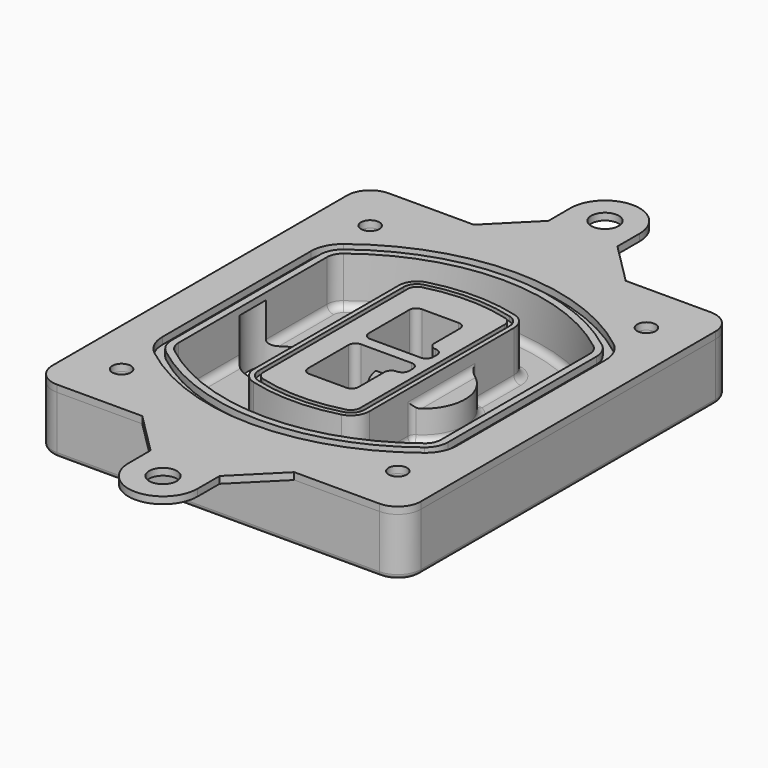
from build123d import *

# Parameters (mm, degrees)
F0_R      = 4
F1_DEPTH  = 25
F2_DEPTH  = 3
F3_DEPTH  = 18
F5_DEPTH  = 21
F6_DEPTH  = 2
F8_DEPTH  = 20
F9_DEPTH  = 16
F10_DEPTH = 25
F7_R      = 6
F7_R_2    = 4
F11_DEPTH = 6
F13_DEPTH = 9
F14_R     = 3
F15_R     = 2
F16_R     = 6
F16_R_2   = 4
F17_DEPTH = 3


with BuildPart() as f1:
    # F0 (on Top) → F1 (new body)
    with BuildSketch(Plane.XY):
        with BuildLine():
            ThreePointArc((-80, -80), (-77.0710678119, -87.0710678119), (-70, -90))
            Line((-70, -90), (70, -90))
            ThreePointArc((70, -90), (77.0710678119, -87.0710678119), (80, -80))
            Line((80, -80), (80, 80))
            ThreePointArc((80, 80), (77.0710678119, 87.0710678119), (70, 90))
            Line((70, 90), (-70, 90))
            ThreePointArc((-70, 90), (-77.0710678119, 87.0710678119), (-80, 80))
            Line((-80, 80), (-80, -80))
        make_face()
        with Locations((-60, -67.5)):
            Circle(F0_R, mode=Mode.SUBTRACT)
        with Locations((60, -67.5)):
            Circle(F0_R, mode=Mode.SUBTRACT)
        with Locations((-60, 67.5)):
            Circle(F0_R, mode=Mode.SUBTRACT)
        with BuildLine():
            ThreePointArc((-64, 40.2934422872), (-62.5820384798, 46.4328484224), (-58.6153846154, 51.3286200352))
            ThreePointArc((-58.6153846154, 51.3286200352), (0, 71.5), (58.6153846154, 51.3286200352))
            ThreePointArc((58.6153846154, 51.3286200352), (62.5820384798, 46.4328484224), (64, 40.2934422872))
            Line((64, 40.2934422872), (64, -40.2934422872))
            ThreePointArc((64, -40.2934422872), (62.5820384798, -46.4328484224), (58.6153846154, -51.3286200352))
            ThreePointArc((58.6153846154, -51.3286200352), (0, -71.5), (-58.6153846154, -51.3286200352))
            ThreePointArc((-58.6153846154, -51.3286200352), (-62.5820384798, -46.4328484224), (-64, -40.2934422872))
            Line((-64, -40.2934422872), (-64, 40.2934422872))
        make_face(mode=Mode.SUBTRACT)
        with Locations((60, 67.5)):
            Circle(F0_R, mode=Mode.SUBTRACT)
        with BuildLine():
            ThreePointArc((58.6153846154, 51.3286200352), (0, 71.5), (-58.6153846154, 51.3286200352))
            ThreePointArc((-58.6153846154, 51.3286200352), (-62.5820384798, 46.4328484224), (-64, 40.2934422872))
            Line((-64, 40.2934422872), (-64, -40.2934422872))
            ThreePointArc((-64, -40.2934422872), (-62.5820384798, -46.4328484224), (-58.6153846154, -51.3286200352))
            ThreePointArc((-58.6153846154, -51.3286200352), (0, -71.5), (58.6153846154, -51.3286200352))
            ThreePointArc((58.6153846154, -51.3286200352), (62.5820384798, -46.4328484224), (64, -40.2934422872))
            Line((64, -40.2934422872), (64, 40.2934422872))
            ThreePointArc((64, 40.2934422872), (62.5820384798, 46.4328484224), (58.6153846154, 51.3286200352))
        make_face()
        with BuildLine():
            Line((-60, -40.2934422872), (-60, 40.2934422872))
            ThreePointArc((-60, 40.2934422872), (-58.9871703427, 44.6787323838), (-56.1538461538, 48.1757121072))
            ThreePointArc((-56.1538461538, 48.1757121072), (0, 67.5), (56.1538461538, 48.1757121072))
            ThreePointArc((56.1538461538, 48.1757121072), (58.9871703427, 44.6787323838), (60, 40.2934422872))
            Line((60, 40.2934422872), (60, -40.2934422872))
            ThreePointArc((60, -40.2934422872), (58.9871703427, -44.6787323838), (56.1538461538, -48.1757121072))
            ThreePointArc((56.1538461538, -48.1757121072), (0, -67.5), (-56.1538461538, -48.1757121072))
            ThreePointArc((-56.1538461538, -48.1757121072), (-58.9871703427, -44.6787323838), (-60, -40.2934422872))
        make_face(mode=Mode.SUBTRACT)
        with BuildLine():
            ThreePointArc((-56.1538461538, 48.1757121072), (-58.9871703427, 44.6787323838), (-60, 40.2934422872))
            Line((-60, 40.2934422872), (-60, -40.2934422872))
            ThreePointArc((-60, -40.2934422872), (-58.9871703427, -44.6787323838), (-56.1538461538, -48.1757121072))
            ThreePointArc((-56.1538461538, -48.1757121072), (0, -67.5), (56.1538461538, -48.1757121072))
            ThreePointArc((56.1538461538, -48.1757121072), (58.9871703427, -44.6787323838), (60, -40.2934422872))
            Line((60, -40.2934422872), (60, 40.2934422872))
            ThreePointArc((60, 40.2934422872), (58.9871703427, 44.6787323838), (56.1538461538, 48.1757121072))
            ThreePointArc((56.1538461538, 48.1757121072), (0, 67.5), (-56.1538461538, 48.1757121072))
        make_face()
        with BuildLine():
            ThreePointArc((54.3076923077, 45.8110311612), (56.2910192399, 43.3631453548), (57, 40.2934422872))
            Line((57, 40.2934422872), (57, -40.2934422872))
            ThreePointArc((57, -40.2934422872), (56.2910192399, -43.3631453548), (54.3076923077, -45.8110311612))
            ThreePointArc((54.3076923077, -45.8110311612), (0, -64.5), (-54.3076923077, -45.8110311612))
            ThreePointArc((-54.3076923077, -45.8110311612), (-56.2910192399, -43.3631453548), (-57, -40.2934422872))
            Line((-57, -40.2934422872), (-57, 40.2934422872))
            ThreePointArc((-57, 40.2934422872), (-56.2910192399, 43.3631453548), (-54.3076923077, 45.8110311612))
            ThreePointArc((-54.3076923077, 45.8110311612), (0, 64.5), (54.3076923077, 45.8110311612))
        make_face(mode=Mode.SUBTRACT)
        with BuildLine():
            Line((57, -40.2934422872), (57, 40.2934422872))
            ThreePointArc((57, 40.2934422872), (56.2910192399, 43.3631453548), (54.3076923077, 45.8110311612))
            ThreePointArc((54.3076923077, 45.8110311612), (0, 64.5), (-54.3076923077, 45.8110311612))
            ThreePointArc((-54.3076923077, 45.8110311612), (-56.2910192399, 43.3631453548), (-57, 40.2934422872))
            Line((-57, 40.2934422872), (-57, -40.2934422872))
            ThreePointArc((-57, -40.2934422872), (-56.2910192399, -43.3631453548), (-54.3076923077, -45.8110311612))
            ThreePointArc((-54.3076923077, -45.8110311612), (0, -64.5), (54.3076923077, -45.8110311612))
            ThreePointArc((54.3076923077, -45.8110311612), (56.2910192399, -43.3631453548), (57, -40.2934422872))
        make_face()
    extrude(amount=-F1_DEPTH)

    # F0 (on Top) → F2 (join)
    with BuildSketch(Plane.XY):
        with BuildLine():
            ThreePointArc((-56.1538461538, 48.1757121072), (-58.9871703427, 44.6787323838), (-60, 40.2934422872))
            Line((-60, 40.2934422872), (-60, -40.2934422872))
            ThreePointArc((-60, -40.2934422872), (-58.9871703427, -44.6787323838), (-56.1538461538, -48.1757121072))
            ThreePointArc((-56.1538461538, -48.1757121072), (0, -67.5), (56.1538461538, -48.1757121072))
            ThreePointArc((56.1538461538, -48.1757121072), (58.9871703427, -44.6787323838), (60, -40.2934422872))
            Line((60, -40.2934422872), (60, 40.2934422872))
            ThreePointArc((60, 40.2934422872), (58.9871703427, 44.6787323838), (56.1538461538, 48.1757121072))
            ThreePointArc((56.1538461538, 48.1757121072), (0, 67.5), (-56.1538461538, 48.1757121072))
        make_face()
        with BuildLine():
            ThreePointArc((54.3076923077, 45.8110311612), (56.2910192399, 43.3631453548), (57, 40.2934422872))
            Line((57, 40.2934422872), (57, -40.2934422872))
            ThreePointArc((57, -40.2934422872), (56.2910192399, -43.3631453548), (54.3076923077, -45.8110311612))
            ThreePointArc((54.3076923077, -45.8110311612), (0, -64.5), (-54.3076923077, -45.8110311612))
            ThreePointArc((-54.3076923077, -45.8110311612), (-56.2910192399, -43.3631453548), (-57, -40.2934422872))
            Line((-57, -40.2934422872), (-57, 40.2934422872))
            ThreePointArc((-57, 40.2934422872), (-56.2910192399, 43.3631453548), (-54.3076923077, 45.8110311612))
            ThreePointArc((-54.3076923077, 45.8110311612), (0, 64.5), (54.3076923077, 45.8110311612))
        make_face(mode=Mode.SUBTRACT)
    extrude(amount=F2_DEPTH)

    # F0 (on Top) → F3 (cut)
    with BuildSketch(Plane.XY):
        with BuildLine():
            Line((57, -40.2934422872), (57, 40.2934422872))
            ThreePointArc((57, 40.2934422872), (56.2910192399, 43.3631453548), (54.3076923077, 45.8110311612))
            ThreePointArc((54.3076923077, 45.8110311612), (0, 64.5), (-54.3076923077, 45.8110311612))
            ThreePointArc((-54.3076923077, 45.8110311612), (-56.2910192399, 43.3631453548), (-57, 40.2934422872))
            Line((-57, 40.2934422872), (-57, -40.2934422872))
            ThreePointArc((-57, -40.2934422872), (-56.2910192399, -43.3631453548), (-54.3076923077, -45.8110311612))
            ThreePointArc((-54.3076923077, -45.8110311612), (0, -64.5), (54.3076923077, -45.8110311612))
            ThreePointArc((54.3076923077, -45.8110311612), (56.2910192399, -43.3631453548), (57, -40.2934422872))
        make_face()
    extrude(amount=-F3_DEPTH, mode=Mode.SUBTRACT)

    # F4 (on face) → F5 (join, through all)
    with BuildSketch(Plane.XY.offset(3)):
        with BuildLine():
            ThreePointArc((-25, -39.2465276821), (-23.3511545998, -44.1109737193), (-19.0842911877, -46.9702398883))
            ThreePointArc((-19.0842911877, -46.9702398883), (0, -49.5), (19.0842911877, -46.9702398883))
            ThreePointArc((19.0842911877, -46.9702398883), (23.3511545998, -44.1109737193), (25, -39.2465276821))
            Line((25, -39.2465276821), (25, 39.2465276821))
            ThreePointArc((25, 39.2465276821), (23.3511545998, 44.1109737193), (19.0842911877, 46.9702398883))
            ThreePointArc((19.0842911877, 46.9702398883), (0, 49.5), (-19.0842911877, 46.9702398883))
            ThreePointArc((-19.0842911877, 46.9702398883), (-23.3511545998, 44.1109737193), (-25, 39.2465276821))
            Line((-25, 39.2465276821), (-25, -39.2465276821))
        make_face()
        with BuildLine():
            ThreePointArc((18.5632183908, 45.0393118368), (21.7633659499, 42.89486221), (23, 39.2465276821))
            Line((23, 39.2465276821), (23, -39.2465276821))
            ThreePointArc((23, -39.2465276821), (21.7633659499, -42.89486221), (18.5632183908, -45.0393118368))
            ThreePointArc((18.5632183908, -45.0393118368), (0, -47.5), (-18.5632183908, -45.0393118368))
            ThreePointArc((-18.5632183908, -45.0393118368), (-21.7633659499, -42.89486221), (-23, -39.2465276821))
            Line((-23, -39.2465276821), (-23, 39.2465276821))
            ThreePointArc((-23, 39.2465276821), (-21.7633659499, 42.89486221), (-18.5632183908, 45.0393118368))
            ThreePointArc((-18.5632183908, 45.0393118368), (0, 47.5), (18.5632183908, 45.0393118368))
        make_face(mode=Mode.SUBTRACT)
        with BuildLine():
            Line((23, -39.2465276821), (23, 39.2465276821))
            ThreePointArc((23, 39.2465276821), (21.7633659499, 42.89486221), (18.5632183908, 45.0393118368))
            ThreePointArc((18.5632183908, 45.0393118368), (0, 47.5), (-18.5632183908, 45.0393118368))
            ThreePointArc((-18.5632183908, 45.0393118368), (-21.7633659499, 42.89486221), (-23, 39.2465276821))
            Line((-23, 39.2465276821), (-23, -39.2465276821))
            ThreePointArc((-23, -39.2465276821), (-21.7633659499, -42.89486221), (-18.5632183908, -45.0393118368))
            ThreePointArc((-18.5632183908, -45.0393118368), (0, -47.5), (18.5632183908, -45.0393118368))
            ThreePointArc((18.5632183908, -45.0393118368), (21.7633659499, -42.89486221), (23, -39.2465276821))
        make_face()
        with BuildLine():
            ThreePointArc((18.0421455939, 43.1083837852), (20.1755772999, 41.6787507007), (21, 39.2465276821))
            Line((21, 39.2465276821), (21, -39.2465276821))
            ThreePointArc((21, -39.2465276821), (20.1755772999, -41.6787507007), (18.0421455939, -43.1083837852))
            ThreePointArc((18.0421455939, -43.1083837852), (0, -45.5), (-18.0421455939, -43.1083837852))
            ThreePointArc((-18.0421455939, -43.1083837852), (-20.1755772999, -41.6787507007), (-21, -39.2465276821))
            Line((-21, -39.2465276821), (-21, 39.2465276821))
            ThreePointArc((-21, 39.2465276821), (-20.1755772999, 41.6787507007), (-18.0421455939, 43.1083837852))
            ThreePointArc((-18.0421455939, 43.1083837852), (0, 45.5), (18.0421455939, 43.1083837852))
        make_face(mode=Mode.SUBTRACT)
        with BuildLine():
            Line((21, -39.2465276821), (21, 39.2465276821))
            ThreePointArc((21, 39.2465276821), (20.1755772999, 41.6787507007), (18.0421455939, 43.1083837852))
            ThreePointArc((18.0421455939, 43.1083837852), (0, 45.5), (-18.0421455939, 43.1083837852))
            ThreePointArc((-18.0421455939, 43.1083837852), (-20.1755772999, 41.6787507007), (-21, 39.2465276821))
            Line((-21, 39.2465276821), (-21, -39.2465276821))
            ThreePointArc((-21, -39.2465276821), (-20.1755772999, -41.6787507007), (-18.0421455939, -43.1083837852))
            ThreePointArc((-18.0421455939, -43.1083837852), (0, -45.5), (18.0421455939, -43.1083837852))
            ThreePointArc((18.0421455939, -43.1083837852), (20.1755772999, -41.6787507007), (21, -39.2465276821))
        make_face()
        with BuildLine():
            Line((-8, -2.5), (14, -2.5))
            ThreePointArc((14, -2.5), (16.1213203436, -3.3786796564), (17, -5.5))
            Line((17, -5.5), (17, -7.5))
            ThreePointArc((17, -7.5), (16.1213203436, -9.6213203436), (14, -10.5))
            ThreePointArc((14, -10.5), (11.8786796564, -11.3786796564), (11, -13.5))
            Line((11, -13.5), (11, -27.5))
            ThreePointArc((11, -27.5), (10.1213203436, -29.6213203436), (8, -30.5))
            Line((8, -30.5), (-8, -30.5))
            ThreePointArc((-8, -30.5), (-10.1213203436, -29.6213203436), (-11, -27.5))
            Line((-11, -27.5), (-11, -5.5))
            ThreePointArc((-11, -5.5), (-10.1213203436, -3.3786796564), (-8, -2.5))
        make_face(mode=Mode.SUBTRACT)
        with BuildLine():
            ThreePointArc((-8, 2.5), (-10.1213203436, 3.3786796564), (-11, 5.5))
            Line((-11, 5.5), (-11, 27.5))
            ThreePointArc((-11, 27.5), (-10.1213203436, 29.6213203436), (-8, 30.5))
            Line((-8, 30.5), (8, 30.5))
            ThreePointArc((8, 30.5), (10.1213203436, 29.6213203436), (11, 27.5))
            Line((11, 27.5), (11, 13.5))
            ThreePointArc((11, 13.5), (11.8786796564, 11.3786796564), (14, 10.5))
            ThreePointArc((14, 10.5), (16.1213203436, 9.6213203436), (17, 7.5))
            Line((17, 7.5), (17, 5.5))
            ThreePointArc((17, 5.5), (16.1213203436, 3.3786796564), (14, 2.5))
            Line((14, 2.5), (-8, 2.5))
        make_face(mode=Mode.SUBTRACT)
    extrude(amount=-F5_DEPTH)

    # F4 (on face) → F6 (cut)
    with BuildSketch(Plane.XY.offset(3)):
        with BuildLine():
            Line((23, -39.2465276821), (23, 39.2465276821))
            ThreePointArc((23, 39.2465276821), (21.7633659499, 42.89486221), (18.5632183908, 45.0393118368))
            ThreePointArc((18.5632183908, 45.0393118368), (0, 47.5), (-18.5632183908, 45.0393118368))
            ThreePointArc((-18.5632183908, 45.0393118368), (-21.7633659499, 42.89486221), (-23, 39.2465276821))
            Line((-23, 39.2465276821), (-23, -39.2465276821))
            ThreePointArc((-23, -39.2465276821), (-21.7633659499, -42.89486221), (-18.5632183908, -45.0393118368))
            ThreePointArc((-18.5632183908, -45.0393118368), (0, -47.5), (18.5632183908, -45.0393118368))
            ThreePointArc((18.5632183908, -45.0393118368), (21.7633659499, -42.89486221), (23, -39.2465276821))
        make_face()
        with BuildLine():
            ThreePointArc((18.0421455939, 43.1083837852), (20.1755772999, 41.6787507007), (21, 39.2465276821))
            Line((21, 39.2465276821), (21, -39.2465276821))
            ThreePointArc((21, -39.2465276821), (20.1755772999, -41.6787507007), (18.0421455939, -43.1083837852))
            ThreePointArc((18.0421455939, -43.1083837852), (0, -45.5), (-18.0421455939, -43.1083837852))
            ThreePointArc((-18.0421455939, -43.1083837852), (-20.1755772999, -41.6787507007), (-21, -39.2465276821))
            Line((-21, -39.2465276821), (-21, 39.2465276821))
            ThreePointArc((-21, 39.2465276821), (-20.1755772999, 41.6787507007), (-18.0421455939, 43.1083837852))
            ThreePointArc((-18.0421455939, 43.1083837852), (0, 45.5), (18.0421455939, 43.1083837852))
        make_face(mode=Mode.SUBTRACT)
    extrude(amount=-F6_DEPTH, mode=Mode.SUBTRACT)

    # F7 (on face) → F8 (join)
    with BuildSketch(Plane(origin=(0, 0, -25), x_dir=(1, 0, 0), z_dir=(0, 0, -1))):
        with BuildLine():
            ThreePointArc((3.28842436, 0), (16.7567035675, 13.4682792075), (30.224982775, 0))
            Line((30.224982775, 0), (35.224982775, 0))
            ThreePointArc((35.224982775, 0), (16.7567035675, 18.4682792075), (-1.71157564, 0))
            Line((-1.71157564, 0), (3.28842436, 0))
        make_face()
        with BuildLine():
            Line((3.28842436, 0), (30.224982775, 0))
            ThreePointArc((30.224982775, 0), (16.7567035675, 13.4682792075), (3.28842436, 0))
        make_face()
        with BuildLine():
            ThreePointArc((3.28842436, 0), (16.7567035675, -13.4682792075), (30.224982775, 0))
            Line((30.224982775, 0), (3.28842436, 0))
        make_face()
        with BuildLine():
            Line((35.224982775, 0), (30.224982775, 0))
            ThreePointArc((30.224982775, 0), (16.7567035675, -13.4682792075), (3.28842436, 0))
            Line((3.28842436, 0), (-1.71157564, 0))
            ThreePointArc((-1.71157564, 0), (16.7567035675, -18.4682792075), (35.224982775, 0))
        make_face()
    extrude(amount=-F8_DEPTH)

    # F7 (on face) → F9 (cut)
    with BuildSketch(Plane(origin=(0, 0, -25), x_dir=(1, 0, 0), z_dir=(0, 0, -1))):
        with BuildLine():
            Line((3.28842436, 0), (30.224982775, 0))
            ThreePointArc((30.224982775, 0), (16.7567035675, 13.4682792075), (3.28842436, 0))
        make_face()
        with BuildLine():
            ThreePointArc((3.28842436, 0), (16.7567035675, -13.4682792075), (30.224982775, 0))
            Line((30.224982775, 0), (3.28842436, 0))
        make_face()
    extrude(amount=-F9_DEPTH, mode=Mode.SUBTRACT)

    # F7 (on face) → F10 (cut)
    with BuildSketch(Plane(origin=(0, 0, -25), x_dir=(1, 0, 0), z_dir=(0, 0, -1))):
        with BuildLine():
            Line((-59.0318229325, 0), (-32.0952645175, 0))
            ThreePointArc((-32.0952645175, 0), (-45.563543725, 13.4682792075), (-59.0318229325, 0))
        make_face()
        with BuildLine():
            ThreePointArc((-59.0318229325, 0), (-45.563543725, -13.4682792075), (-32.0952645175, 0))
            Line((-32.0952645175, 0), (-59.0318229325, 0))
        make_face()
    extrude(amount=-F10_DEPTH, mode=Mode.SUBTRACT)

    # F7 (on face) → F11 (cut)
    with BuildSketch(Plane(origin=(0, 0, -25), x_dir=(1, 0, 0), z_dir=(0, 0, -1))):
        with Locations((60, -67.5)):
            Circle(F7_R)
        with Locations((60, -67.5)):
            Circle(F7_R_2, mode=Mode.SUBTRACT)
        with Locations((-60, -67.5)):
            Circle(F7_R)
        with Locations((-60, -67.5)):
            Circle(F7_R_2, mode=Mode.SUBTRACT)
        with Locations((-60, 67.5)):
            Circle(F7_R)
        with Locations((-60, 67.5)):
            Circle(F7_R_2, mode=Mode.SUBTRACT)
        with Locations((60, 67.5)):
            Circle(F7_R)
        with Locations((60, 67.5)):
            Circle(F7_R_2, mode=Mode.SUBTRACT)
    extrude(amount=-F11_DEPTH, mode=Mode.SUBTRACT)

    # F12 (on face) → F13 (cut, through all)
    with BuildSketch(Plane(origin=(0, 0, -9), x_dir=(1, 0, 0), z_dir=(0, 0, -1))):
        with BuildLine():
            Line((11, 13.5), (11, 17.5481537753))
            ThreePointArc((11, 17.5481537753), (2.5696536419, 11.8239143813), (-1.5415842455, 2.5))
            Line((-1.5415842455, 2.5), (3.5224848595, 2.5))
            ThreePointArc((3.5224848595, 2.5), (6.1857188154, 8.3455872281), (11.2536447004, 12.2927168648))
            ThreePointArc((11.2536447004, 12.2927168648), (11.0640958889, 12.8831798879), (11, 13.5))
        make_face()
        with BuildLine():
            ThreePointArc((11.2536447004, -12.2927168648), (6.1857188154, -8.3455872281), (3.5224848595, -2.5))
            Line((3.5224848595, -2.5), (-1.5415842455, -2.5))
            ThreePointArc((-1.5415842455, -2.5), (2.5696536419, -11.8239143813), (11, -17.5481537753))
            Line((11, -17.5481537753), (11, -13.5))
            ThreePointArc((11, -13.5), (11.0640958889, -12.8831798879), (11.2536447004, -12.2927168648))
        make_face()
        with BuildLine():
            ThreePointArc((11.2536447004, 12.2927168648), (6.1857188154, 8.3455872281), (3.5224848595, 2.5))
            Line((3.5224848595, 2.5), (14, 2.5))
            ThreePointArc((14, 2.5), (16.1213203436, 3.3786796564), (17, 5.5))
            Line((17, 5.5), (17, 7.5))
            ThreePointArc((17, 7.5), (16.1213203436, 9.6213203436), (14, 10.5))
            ThreePointArc((14, 10.5), (12.3601599782, 10.9878446101), (11.2536447004, 12.2927168648))
        make_face()
        with BuildLine():
            Line((14, -2.5), (3.5224848595, -2.5))
            ThreePointArc((3.5224848595, -2.5), (6.1857188154, -8.3455872281), (11.2536447004, -12.2927168648))
            ThreePointArc((11.2536447004, -12.2927168648), (12.3601599782, -10.9878446101), (14, -10.5))
            ThreePointArc((14, -10.5), (16.1213203436, -9.6213203436), (17, -7.5))
            Line((17, -7.5), (17, -5.5))
            ThreePointArc((17, -5.5), (16.1213203436, -3.3786796564), (14, -2.5))
        make_face()
    extrude(amount=F13_DEPTH, mode=Mode.SUBTRACT)

    # F14
    f14_edges = [f1.edges().sort_by_distance(p)[0] for p in [
        (-57, -23.703476, -18),
        (-57, 23.703476, -18),
        (25, 0, -5),
        (25, 16.526506, -11.5),
        (25, -16.526506, -11.5),
        (25, -27.886517, -18),
        (35.224983, 0, -18),
    ]]
    fillet(f14_edges, radius=F14_R)

    # F15
    f15_edges = [f1.edges().sort_by_distance(p)[0] for p in [
        (0, -90, -25),
    ]]
    fillet(f15_edges, radius=F15_R)


with BuildPart() as f17:
    # F16 (on face) → F17 (new body, through all)
    with BuildSketch(Plane.XY):
        with BuildLine():
            Line((33, -90), (-33, -90))
            Line((-33, -90), (-15, -108))
            Line((-15, -108), (-15, -120))
            ThreePointArc((-15, -120), (0, -135), (15, -120))
            Line((15, -120), (15, -108))
            Line((15, -108), (33, -90))
        make_face()
        with Locations((0, -120)):
            Circle(F16_R, mode=Mode.SUBTRACT)
        with BuildLine():
            Line((33, 90), (-33, 90))
            Line((-33, 90), (-70, 90))
            ThreePointArc((-70, 90), (-77.0710678119, 87.0710678119), (-80, 80))
            Line((-80, 80), (-80, -80))
            ThreePointArc((-80, -80), (-77.0710678119, -87.0710678119), (-70, -90))
            Line((-70, -90), (-33, -90))
            Line((-33, -90), (33, -90))
            Line((33, -90), (70, -90))
            ThreePointArc((70, -90), (77.0710678119, -87.0710678119), (80, -80))
            Line((80, -80), (80, 80))
            ThreePointArc((80, 80), (77.0710678119, 87.0710678119), (70, 90))
            Line((70, 90), (33, 90))
        make_face()
        with Locations((-60, -67.5)):
            Circle(F16_R_2, mode=Mode.SUBTRACT)
        with Locations((60, -67.5)):
            Circle(F16_R_2, mode=Mode.SUBTRACT)
        with Locations((-60, 67.5)):
            Circle(F16_R_2, mode=Mode.SUBTRACT)
        with BuildLine():
            Line((-64, -40.2934422872), (-64, 40.2934422872))
            ThreePointArc((-64, 40.2934422872), (-62.5820384798, 46.4328484224), (-58.6153846154, 51.3286200352))
            ThreePointArc((-58.6153846154, 51.3286200352), (0, 71.5), (58.6153846154, 51.3286200352))
            ThreePointArc((58.6153846154, 51.3286200352), (62.5820384798, 46.4328484224), (64, 40.2934422872))
            Line((64, 40.2934422872), (64, -40.2934422872))
            ThreePointArc((64, -40.2934422872), (62.5820384798, -46.4328484224), (58.6153846154, -51.3286200352))
            ThreePointArc((58.6153846154, -51.3286200352), (0, -71.5), (-58.6153846154, -51.3286200352))
            ThreePointArc((-58.6153846154, -51.3286200352), (-62.5820384798, -46.4328484224), (-64, -40.2934422872))
        make_face(mode=Mode.SUBTRACT)
        with Locations((60, 67.5)):
            Circle(F16_R_2, mode=Mode.SUBTRACT)
        with BuildLine():
            ThreePointArc((15, 120), (0, 135), (-15, 120))
            Line((-15, 120), (-15, 108))
            Line((-15, 108), (-33, 90))
            Line((-33, 90), (33, 90))
            Line((33, 90), (15, 108))
            Line((15, 108), (15, 120))
        make_face()
        with Locations((0, 120)):
            Circle(F16_R, mode=Mode.SUBTRACT)
    extrude(amount=F17_DEPTH)


solid = Compound([f1.part, f17.part])
